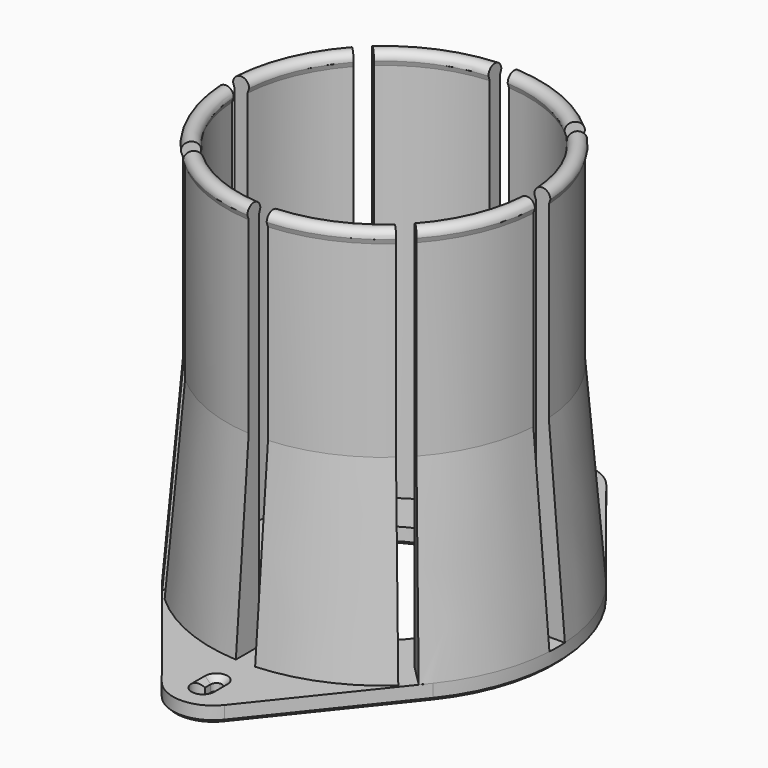
from build123d import *

# Parameters (mm, degrees)
F3_R     = 30
F4_DEPTH = 5
F5_DEPTH = 5
F7_START = 5
F7_DEPTH = 145
F8_SIZE  = 1.74999
F9_SIZE  = 1


# Not quite as in the source:
# - a fillet or chamfer is up to 0.001 mm smaller than in the source, because OpenCascade refuses the exact size
# - a feature names something its author has since deleted; it is built from what else it names


with BuildPart() as f2:
    # F1 (on Front) → F2 (revolve)
    with BuildSketch(Plane.XZ):
        Polygon((-54, 0), (0, 0), (0, 5), (-45, 5), (-49, 5), (-54, 5), align=None)
        Polygon((-49, 65), (-54, 5), (-49, 5), align=None)
        with BuildLine():
            Line((-49, 5), (-45, 5))
            Line((-45, 5), (-45, 123.5))
            ThreePointArc((-45, 123.5), (-47, 122.5), (-49, 123.5))
            Line((-49, 123.5), (-49, 65))
            Line((-49, 65), (-49, 5))
        make_face()
        with BuildLine():
            ThreePointArc((-49, 123.5), (-47, 122.5), (-45, 123.5))
            Line((-45, 123.5), (-44.5, 125))
            ThreePointArc((-44.5, 125), (-47, 127.5), (-49.5, 125))
            Line((-49.5, 125), (-49, 123.5))
        make_face()
    revolve(axis=Axis((0, 0, 56.3952513039), (0, 0, 1)))

    # F3 (on Top) → F4 (join)
    with BuildSketch(Plane.XY):
        with BuildLine():
            Line((42.194320425, 33.6992481203), (9.7672038021, 74.3007518797))
            ThreePointArc((9.7672038021, 74.3007518797), (0, 79), (-9.7672038021, 74.3007518797))
            Line((-9.7672038021, 74.3007518797), (-42.194320425, 33.6992481203))
            ThreePointArc((-42.194320425, 33.6992481203), (-54, 0), (-42.194320425, -33.6992481203))
            Line((-42.194320425, -33.6992481203), (-9.7672038021, -74.3007518797))
            ThreePointArc((-9.7672038021, -74.3007518797), (0, -79), (9.7672038021, -74.3007518797))
            Line((9.7672038021, -74.3007518797), (42.194320425, -33.6992481203))
            ThreePointArc((42.194320425, -33.6992481203), (54, 0), (42.194320425, 33.6992481203))
        make_face()
        with BuildLine():
            ThreePointArc((1.75, -67.4689110868), (3.0310889132, -68.75), (3.5, -70.5))
            ThreePointArc((3.5, -70.5), (-1.75, -73.5310889132), (-1.75, -67.4689110868))
            Line((-1.75, -67.4689110868), (-1.75, -65.25))
            ThreePointArc((-1.75, -65.25), (0, -63.5), (1.75, -65.25))
            Line((1.75, -65.25), (1.75, -67.4689110868))
        make_face(mode=Mode.SUBTRACT)
        Circle(F3_R, mode=Mode.SUBTRACT)
        with BuildLine():
            ThreePointArc((-1.75, 69.25), (0, 71), (1.75, 69.25))
            Line((1.75, 69.25), (1.75, 67.0310889132))
            ThreePointArc((1.75, 67.0310889132), (3.0310889132, 65.75), (3.5, 64))
            ThreePointArc((3.5, 64), (-1.75, 60.9689110868), (-1.75, 67.0310889132))
            Line((-1.75, 67.0310889132), (-1.75, 69.25))
        make_face(mode=Mode.SUBTRACT)
    extrude(amount=F4_DEPTH)

    # F3 (on Top) → F5 (cut)
    with BuildSketch(Plane.XY):
        Circle(F3_R)
    extrude(amount=F5_DEPTH, mode=Mode.SUBTRACT)

    # F6 (on Top) → F7 (cut)
    with BuildSketch(Plane.XY.offset(F7_START)):
        Polygon((3, 6.5355339059), (3, 75), (-3, 75), (-3, 6.5355339059), (0, 3.5355339059), align=None)
        Polygon((65.1931899483, 68.7287238543), (3, 6.5355339059), (3, 3), (6.5355339059, 3), (68.7287238543, 65.1931899483), align=None)
        Polygon((3, 3), (3, 6.5355339059), (0, 3.5355339059), (0.5355339059, 3), align=None)
        Polygon((0, 3.5355339059), (-3, 6.5355339059), (-3, 3), (-0.5355339059, 3), align=None)
        Polygon((-3, 3), (-3, 6.5355339059), (-65.1931899483, 68.7287238543), (-68.7287238543, 65.1931899483), (-6.5355339059, 3), align=None)
        Polygon((6.5355339059, 3), (3, 3), (3, 0.5355339059), (3.5355339059, 0), align=None)
        Polygon((-3, 0.5355339059), (-3, 3), (-6.5355339059, 3), (-3.5355339059, 0), align=None)
        Polygon((75, 3), (6.5355339059, 3), (3.5355339059, 0), (6.5355339059, -3), (75, -3), align=None)
        Polygon((-3.5355339059, 0), (-6.5355339059, 3), (-75, 3), (-75, -3), (-6.5355339059, -3), align=None)
        Polygon((3.5355339059, 0), (3, -0.5355339059), (3, -3), (6.5355339059, -3), align=None)
        Polygon((-3, -3), (-3, -0.5355339059), (-3.5355339059, 0), (-6.5355339059, -3), align=None)
        Polygon((6.5355339059, -3), (3, -3), (3, -6.5355339059), (60.3179938044, -63.8535277103), (63.8535277103, -60.3179938044), align=None)
        Polygon((3, -6.5355339059), (3, -3), (0.5355339059, -3), (0, -3.5355339059), align=None)
        Polygon((-0.5355339059, -3), (-3, -3), (-3, -6.5355339059), (0, -3.5355339059), align=None)
        Polygon((-3, -6.5355339059), (-3, -3), (-6.5355339059, -3), (-63.8535277103, -60.3179938044), (-60.3179938044, -63.8535277103), align=None)
        Polygon((3, -75), (3, -6.5355339059), (0, -3.5355339059), (-3, -6.5355339059), (-3, -75), align=None)
    extrude(amount=F7_DEPTH, mode=Mode.SUBTRACT)

    # F8 (size 1.75 in the source; OpenCascade refuses exactly that, so slightly less here)
    f8_edges = [f2.edges().sort_by_distance(p)[0] for p in [
        (0, 71, 5),
        (0, -63.5, 5),
    ]]
    chamfer(f8_edges, length=F8_SIZE)

    # F9
    f9_edges = [f2.edges().sort_by_distance(p)[0] for p in [
        (-54, 0, 0),
        (-25.980762, -54, 0),
        (-25.980762, 54, 0),
        (0, -79, 0),
        (0, 79, 0),
        (25.980762, -54, 0),
        (25.980762, 54, 0),
        (54, 0, 0),
        (1.75, 68.140544, 0),
        (0, 71, 0),
        (0, 60.5, 0),
        (-1.75, 68.140544, 0),
        (-30, 0, 0),
        (1.75, -66.359456, 0),
        (0, -63.5, 0),
        (0, -74, 0),
        (-1.75, -66.359456, 0),
    ]]
    chamfer(f9_edges, length=F9_SIZE)


solid = f2.part
